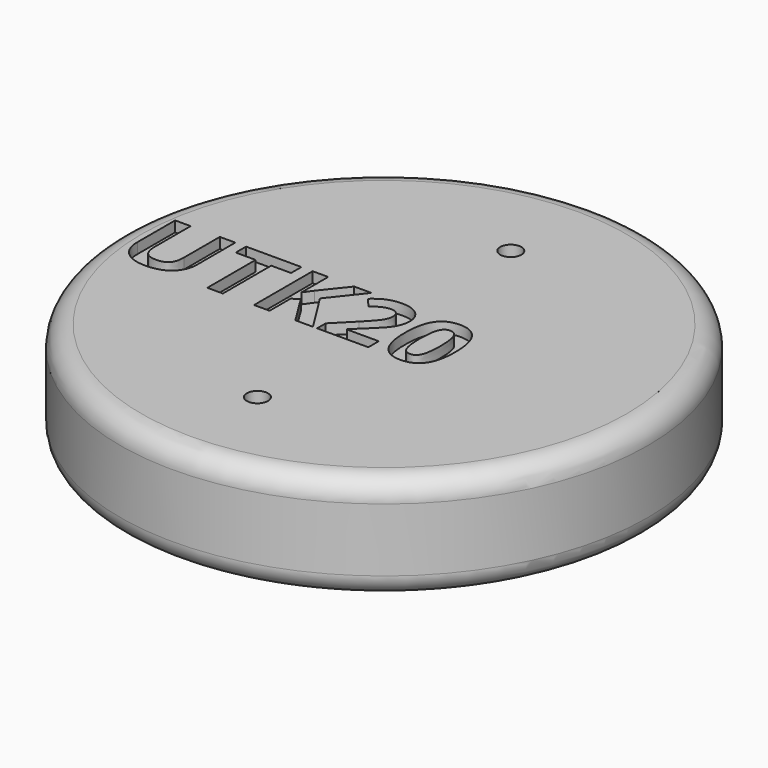
from build123d import *

# Parameters (mm, degrees)
F0_R           = 25
F1_DEPTH       = 10
F2_TEXT_SIZE   = 9.7222222222
F3_DEPTH       = 1
F4_R           = 2
F6_D           = 2
F6_CBORE_D     = 5
F6_CBORE_DEPTH = 2.5


# Not quite as in the source:
# - Text() gives the source's letters only with a copy of the font that has no kerning and outlines rounded to 1/6400 em; it was checked with that copy


with BuildPart() as f1:
    # F0 (on Top) → F1 (new body)
    with BuildSketch(Plane.XY):
        Circle(F0_R)
    extrude(amount=F1_DEPTH)

    # F2 (on face) → F3 (cut)
    with BuildSketch(Plane.XY.offset(10)):
        with Locations((-23.2602746329, -3.6353966245)):
            Text('UTK20', F2_TEXT_SIZE, font='Open Sans', font_style=FontStyle.BOLD, text_align=(TextAlign.LEFT, TextAlign.BOTTOM))
    extrude(amount=-F3_DEPTH, mode=Mode.SUBTRACT)

    # F4
    f4_edges = [f1.edges().sort_by_distance(p)[0] for p in [
        (-25, 0, 10),
        (-25, 0, 0),
    ]]
    fillet(f4_edges, radius=F4_R)

    # F6 (through all)
    with Locations(Plane(origin=(0, 0, 0), x_dir=(1, 0, 0), z_dir=(0, 0, -1))):
        with Locations((0, 15), (0, -15)):
            CounterBoreHole(F6_D / 2, F6_CBORE_D / 2, F6_CBORE_DEPTH)


solid = f1.part
